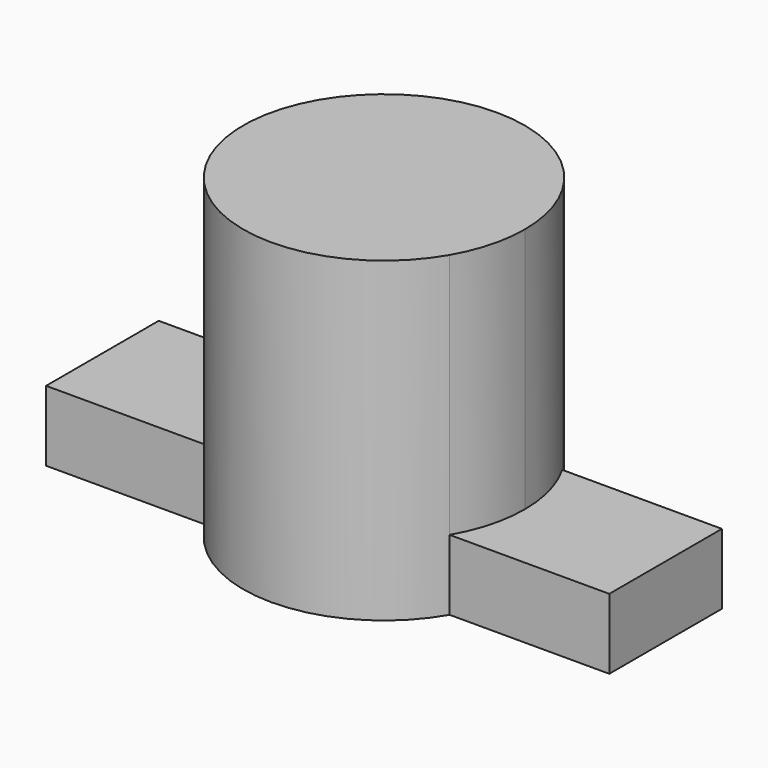
from build123d import *

# Parameters (mm, degrees)
F1_DEPTH = 9
F2_DEPTH = 2


with BuildPart() as f1:
    # F0 (on Top) → F1 (new body)
    with BuildSketch(Plane.XY):
        with BuildLine():
            ThreePointArc((3.4640958416, -2), (3.863698102, -1.0352762805), (3.999995, 0))
            ThreePointArc((3.999995, 0), (3.863698102, 1.0352762805), (3.4640958416, 2))
            Line((3.4640958416, 2), (-3.4640958416, 2))
            ThreePointArc((-3.4640958416, 2), (-3.999995, 0), (-3.4640958416, -2))
            Line((-3.4640958416, -2), (3.4640958416, -2))
        make_face()
        with BuildLine():
            Line((-3.4640958416, 2), (3.4640958416, 2))
            ThreePointArc((3.4640958416, 2), (0, 3.999995), (-3.4640958416, 2))
        make_face()
        with BuildLine():
            ThreePointArc((-3.4640958416, -2), (0, -3.999995), (3.4640958416, -2))
            Line((3.4640958416, -2), (-3.4640958416, -2))
        make_face()
    extrude(amount=F1_DEPTH)

    # F0 (on Top) → F2 (join)
    with BuildSketch(Plane.XY):
        with BuildLine():
            ThreePointArc((3.4640958416, -2), (3.863698102, -1.0352762805), (3.999995, 0))
            ThreePointArc((3.999995, 0), (3.863698102, 1.0352762805), (3.4640958416, 2))
            Line((3.4640958416, 2), (-3.4640958416, 2))
            ThreePointArc((-3.4640958416, 2), (-3.999995, 0), (-3.4640958416, -2))
            Line((-3.4640958416, -2), (3.4640958416, -2))
        make_face()
        with BuildLine():
            ThreePointArc((3.4640958416, 2), (3.863698102, 1.0352762805), (3.999995, 0))
            ThreePointArc((3.999995, 0), (3.863698102, -1.0352762805), (3.4640958416, -2))
            Line((3.4640958416, -2), (8, -2))
            Line((8, -2), (8, 2))
            Line((8, 2), (3.4640958416, 2))
        make_face()
        with BuildLine():
            Line((-3.4640958416, 2), (3.4640958416, 2))
            ThreePointArc((3.4640958416, 2), (0, 3.999995), (-3.4640958416, 2))
        make_face()
        with BuildLine():
            ThreePointArc((-3.4640958416, -2), (0, -3.999995), (3.4640958416, -2))
            Line((3.4640958416, -2), (-3.4640958416, -2))
        make_face()
        with BuildLine():
            ThreePointArc((-3.4640958416, -2), (-3.999995, 0), (-3.4640958416, 2))
            Line((-3.4640958416, 2), (-8, 2))
            Line((-8, 2), (-8, -2))
            Line((-8, -2), (-3.4640958416, -2))
        make_face()
    extrude(amount=F2_DEPTH)


solid = f1.part
